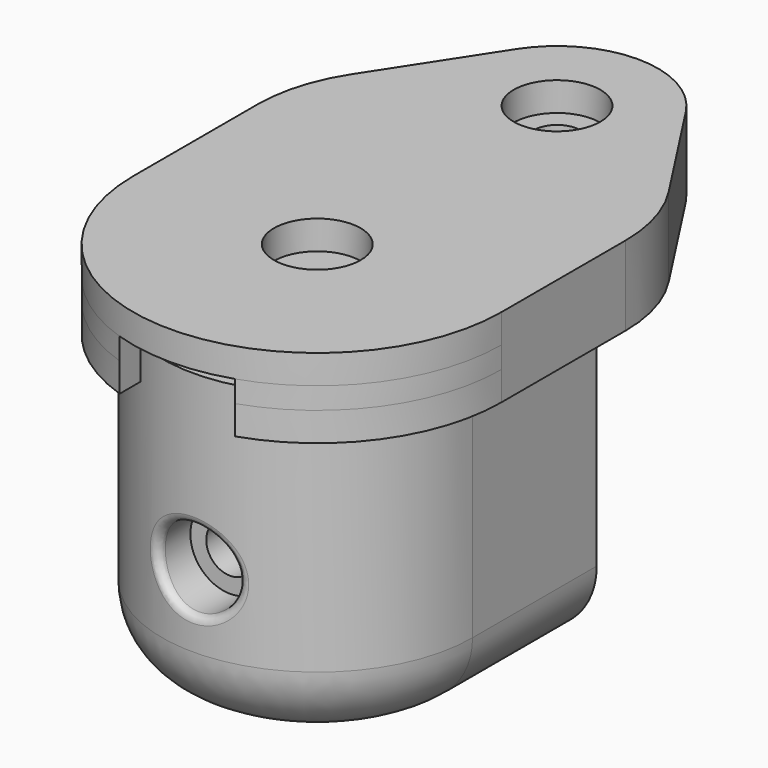
from build123d import *

# Parameters (mm, degrees)
F1_DEPTH  = 20
F2_R      = 1.6
F3_DEPTH  = 2
F4_R      = 1.65
F5_DEPTH  = 30
F8_R      = 2.75
F9_DEPTH  = 3.2
F10_R     = 0.5
F11_R     = 5
F13_DEPTH = 2
F14_R     = 1.6
F15_DEPTH = 1.5
F16_R     = 3
F17_DEPTH = 2
F18_W     = 8
F18_H     = 4.8582903781
F19_DEPTH = 2


# Not quite as in the source:
# - a feature names something its author has since deleted; it is built from what else it names


with BuildPart() as f1:
    # F0 (on Top) → F1 (new body)
    with BuildSketch(Plane.XY):
        with BuildLine():
            Line((10.75, 10.75), (-10.75, 10.75))
            Line((-10.75, 10.75), (-10.75, 0))
            ThreePointArc((-10.75, 0), (0, -10.75), (10.75, 0))
            Line((10.75, 0), (10.75, 10.75))
        make_face()
    extrude(amount=-F1_DEPTH)

    # F2 (on face) → F3 (join)
    with BuildSketch(Plane.XY):
        with BuildLine():
            Line((-10.75, 10.75), (-10.75, 0))
            ThreePointArc((-10.75, 0), (0, -10.75), (10.75, 0))
            Line((10.75, 0), (10.75, 10.75))
            ThreePointArc((10.75, 10.75), (10.383601773, 13.2755372984), (9.3146181955, 15.5928332263))
            Line((9.3146181955, 15.5928332263), (4.1924539291, 23.4745788761))
            ThreePointArc((4.1924539291, 23.4745788761), (0, 25.75), (-4.1924539291, 23.4745788761))
            Line((-4.1924539291, 23.4745788761), (-9.3146181955, 15.5928332263))
            ThreePointArc((-9.3146181955, 15.5928332263), (-10.383601773, 13.2755372984), (-10.75, 10.75))
        make_face()
        with Locations((0, 20.75)):
            Circle(F2_R, mode=Mode.SUBTRACT)
    extrude(amount=F3_DEPTH)

    # F4 (on face) → F5 (cut)
    with BuildSketch(Plane(origin=(0, 10.75, 0), x_dir=(-1, 0, 0), z_dir=(0, 1, 0))):
        with Locations((0, -10)):
            Circle(F4_R)
    extrude(amount=-F5_DEPTH, mode=Mode.SUBTRACT)

    # F8 (on plane+point) → F9 (cut)
    with BuildSketch(Plane.XZ.offset(10.75)):
        with Locations((0, -10)):
            Circle(F8_R)
    extrude(amount=-F9_DEPTH, mode=Mode.SUBTRACT)

    # F10
    f10_edges = [f1.edges().sort_by_distance(p)[0] for p in [
        (-2.749989, -10.392308, -9.992207),
    ]]
    fillet(f10_edges, radius=F10_R)

    # F11
    f11_edges = [f1.edges().sort_by_distance(p)[0] for p in [
        (0, -10.75, -20),
        (10.75, 5.375, -20),
        (-10.75, 5.375, -20),
    ]]
    fillet(f11_edges, radius=F11_R)


with BuildPart() as f13:
    # F12 (on Top) → F13 (new body)
    with BuildSketch(Plane.XY):
        with BuildLine():
            Line((-12.75, 10.75), (-12.75, 0))
            ThreePointArc((-12.75, 0), (0, -12.75), (12.75, 0))
            Line((12.75, 0), (12.75, 10.75))
            ThreePointArc((12.75, 10.75), (12.3011474886, 13.8438844004), (10.9915997671, 16.6826647767))
            Line((10.9915997671, 16.6826647767), (5.8694355008, 24.5644104265))
            ThreePointArc((5.8694355008, 24.5644104265), (0, 27.75), (-5.8694355008, 24.5644104265))
            Line((-5.8694355008, 24.5644104265), (-10.9915997671, 16.6826647767))
            ThreePointArc((-10.9915997671, 16.6826647767), (-12.3011474886, 13.8438844004), (-12.75, 10.75))
        make_face()
        with BuildLine():
            ThreePointArc((11.05, 0), (0, -11.05), (-11.05, 0))
            Line((-11.05, 0), (-11.05, 10.75))
            ThreePointArc((-11.05, 10.75), (-10.6712336303, 13.3607893637), (-9.5661654312, 15.7563079588))
            Line((-9.5661654312, 15.7563079588), (-4.4440011649, 23.6380536087))
            ThreePointArc((-4.4440011649, 23.6380536087), (0, 26.05), (4.4440011649, 23.6380536087))
            Line((4.4440011649, 23.6380536087), (9.5661654312, 15.7563079588))
            ThreePointArc((9.5661654312, 15.7563079588), (10.6712336303, 13.3607893637), (11.05, 10.75))
            Line((11.05, 10.75), (11.05, 0))
        make_face(mode=Mode.SUBTRACT)
    extrude(amount=F13_DEPTH)

    # F14 (on face) → F15 (join)
    with BuildSketch(Plane.XY.offset(2)):
        with BuildLine():
            Line((10.9915997671, 16.6826647767), (5.8694355008, 24.5644104265))
            ThreePointArc((5.8694355008, 24.5644104265), (0, 27.75), (-5.8694355008, 24.5644104265))
            Line((-5.8694355008, 24.5644104265), (-10.9915997671, 16.6826647767))
            ThreePointArc((-10.9915997671, 16.6826647767), (-12.3011474886, 13.8438844004), (-12.75, 10.75))
            Line((-12.75, 10.75), (-12.75, 0))
            ThreePointArc((-12.75, 0), (-10.3335013427, -7.4686846231), (-4, -12.1063000128))
            Line((-4, -12.1063000128), (-4, -8.8917096219))
            ThreePointArc((-4, -8.8917096219), (0, 9.75), (4, -8.8917096219))
            Line((4, -8.8917096219), (4, -12.1063000128))
            ThreePointArc((4, -12.1063000128), (10.3335013427, -7.4686846231), (12.75, 0))
            Line((12.75, 0), (12.75, 10.75))
            ThreePointArc((12.75, 10.75), (12.3011474886, 13.8438844004), (10.9915997671, 16.6826647767))
        make_face()
        with Locations((0, 20.75)):
            Circle(F14_R, mode=Mode.SUBTRACT)
    extrude(amount=F15_DEPTH)

    # F16 (on face) → F17 (join)
    with BuildSketch(Plane.XY.offset(3.5)):
        with BuildLine():
            Line((10.9915997671, 16.6826647767), (5.8694355008, 24.5644104265))
            ThreePointArc((5.8694355008, 24.5644104265), (0, 27.75), (-5.8694355008, 24.5644104265))
            Line((-5.8694355008, 24.5644104265), (-10.9915997671, 16.6826647767))
            ThreePointArc((-10.9915997671, 16.6826647767), (-12.3011474886, 13.8438844004), (-12.75, 10.75))
            Line((-12.75, 10.75), (-12.75, 0))
            ThreePointArc((-12.75, 0), (0, -12.75), (12.75, 0))
            Line((12.75, 0), (12.75, 10.75))
            ThreePointArc((12.75, 10.75), (12.3011474886, 13.8438844004), (10.9915997671, 16.6826647767))
        make_face()
        Circle(F16_R, mode=Mode.SUBTRACT)
        with Locations((0, 20.75)):
            Circle(F16_R, mode=Mode.SUBTRACT)
    extrude(amount=F17_DEPTH)

    # F18 (on face) → F19 (cut, through all)
    with BuildSketch(Plane.XY):
        with Locations((0, -11.3208548109)):
            Rectangle(F18_W, F18_H)
    extrude(amount=F19_DEPTH, mode=Mode.SUBTRACT)


solid = Compound([f1.part, f13.part])
